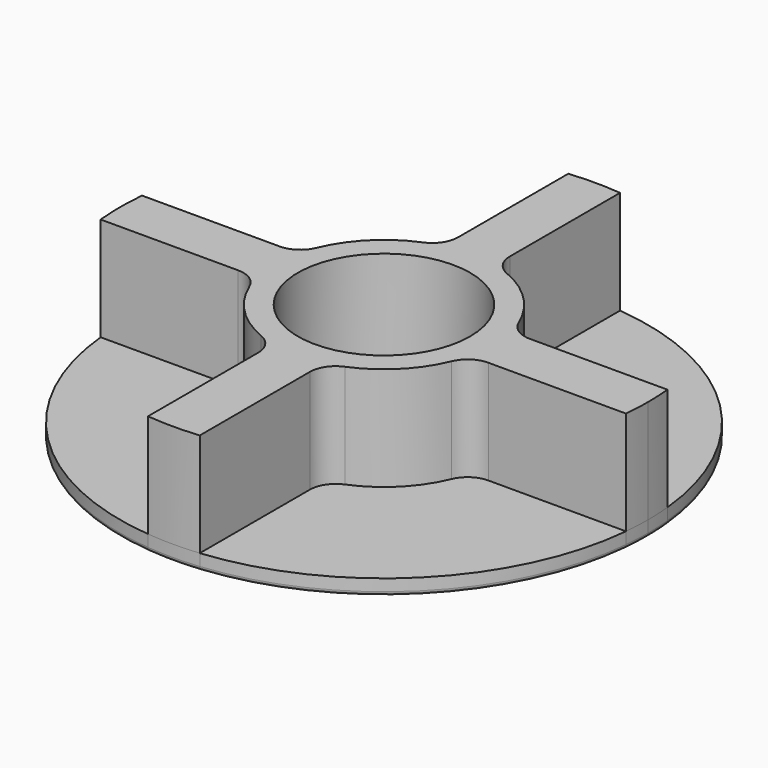
from build123d import *

# Parameters (mm, degrees)
F0_R     = 6.65
F0_R_2   = 1.8
F1_DEPTH = 1.2
F2_DEPTH = 8
F3_R     = 0.3


# Not quite as in the source:
# - a feature names something its author has since deleted; it is built from what else it names


with BuildPart() as f1:
    # F0 (on Top) → F1 (new body)
    with BuildSketch(Plane.XY):
        with BuildLine():
            Line((9.6529388756, 1.998378199), (20.2717385681, 1.998378199))
            ThreePointArc((20.2717385681, 1.998378199), (14.4037651328, 14.4037651328), (1.998378199, 20.2717385681))
            Line((1.998378199, 20.2717385681), (1.998378199, 9.6529388756))
            ThreePointArc((1.998378199, 9.6529388756), (2.3354389744, 8.5417984096), (3.2330113343, 7.8051798106))
            ThreePointArc((3.2330113343, 7.8051798106), (5.9738260003, 5.9738260003), (7.8051798106, 3.2330113343))
            ThreePointArc((7.8051798106, 3.2330113343), (8.5417984096, 2.3354389744), (9.6529388756, 1.998378199))
        make_face()
        with BuildLine():
            Line((-1.998378199, 9.6529388756), (-1.998378199, 20.2717385681))
            ThreePointArc((-1.998378199, 20.2717385681), (-14.4037651328, 14.4037651328), (-20.2717385681, 1.998378199))
            Line((-20.2717385681, 1.998378199), (-9.6529388756, 1.998378199))
            ThreePointArc((-9.6529388756, 1.998378199), (-8.5417984096, 2.3354389744), (-7.8051798106, 3.2330113343))
            ThreePointArc((-7.8051798106, 3.2330113343), (-5.9738260003, 5.9738260003), (-3.2330113343, 7.8051798106))
            ThreePointArc((-3.2330113343, 7.8051798106), (-2.3354389744, 8.5417984096), (-1.998378199, 9.6529388756))
        make_face()
        with BuildLine():
            ThreePointArc((-20.2717385681, -1.998378199), (-14.4037651328, -14.4037651328), (-1.998378199, -20.2717385681))
            Line((-1.998378199, -20.2717385681), (-1.998378199, -9.6529388756))
            ThreePointArc((-1.998378199, -9.6529388756), (-2.3354389744, -8.5417984096), (-3.2330113343, -7.8051798106))
            ThreePointArc((-3.2330113343, -7.8051798106), (-5.9738260003, -5.9738260003), (-7.8051798106, -3.2330113343))
            ThreePointArc((-7.8051798106, -3.2330113343), (-8.5417984096, -2.3354389744), (-9.6529388756, -1.998378199))
            Line((-9.6529388756, -1.998378199), (-20.2717385681, -1.998378199))
        make_face()
        with BuildLine():
            ThreePointArc((1.998378199, -20.2717385681), (14.4037651328, -14.4037651328), (20.2717385681, -1.998378199))
            Line((20.2717385681, -1.998378199), (9.6529388756, -1.998378199))
            ThreePointArc((9.6529388756, -1.998378199), (8.5417984096, -2.3354389744), (7.8051798106, -3.2330113343))
            ThreePointArc((7.8051798106, -3.2330113343), (5.9738260003, -5.9738260003), (3.2330113343, -7.8051798106))
            ThreePointArc((3.2330113343, -7.8051798106), (2.3354389744, -8.5417984096), (1.998378199, -9.6529388756))
            Line((1.998378199, -9.6529388756), (1.998378199, -20.2717385681))
        make_face()
        with BuildLine():
            ThreePointArc((20.2717385681, -1.998378199), (20.3454198117, -1.0003962634), (20.37, 0))
            ThreePointArc((20.37, 0), (20.3454198117, 1.0003962634), (20.2717385681, 1.998378199))
            Line((20.2717385681, 1.998378199), (9.6529388756, 1.998378199))
            ThreePointArc((9.6529388756, 1.998378199), (8.5417984096, 2.3354389744), (7.8051798106, 3.2330113343))
            ThreePointArc((7.8051798106, 3.2330113343), (5.9738260003, 5.9738260003), (3.2330113343, 7.8051798106))
            ThreePointArc((3.2330113343, 7.8051798106), (2.3354389744, 8.5417984096), (1.998378199, 9.6529388756))
            Line((1.998378199, 9.6529388756), (1.998378199, 20.2717385681))
            ThreePointArc((1.998378199, 20.2717385681), (0, 20.37), (-1.998378199, 20.2717385681))
            Line((-1.998378199, 20.2717385681), (-1.998378199, 9.6529388756))
            ThreePointArc((-1.998378199, 9.6529388756), (-2.3354389744, 8.5417984096), (-3.2330113343, 7.8051798106))
            ThreePointArc((-3.2330113343, 7.8051798106), (-5.9738260003, 5.9738260003), (-7.8051798106, 3.2330113343))
            ThreePointArc((-7.8051798106, 3.2330113343), (-8.5417984096, 2.3354389744), (-9.6529388756, 1.998378199))
            Line((-9.6529388756, 1.998378199), (-20.2717385681, 1.998378199))
            ThreePointArc((-20.2717385681, 1.998378199), (-20.37, 0), (-20.2717385681, -1.998378199))
            Line((-20.2717385681, -1.998378199), (-9.6529388756, -1.998378199))
            ThreePointArc((-9.6529388756, -1.998378199), (-8.5417984096, -2.3354389744), (-7.8051798106, -3.2330113343))
            ThreePointArc((-7.8051798106, -3.2330113343), (-5.9738260003, -5.9738260003), (-3.2330113343, -7.8051798106))
            ThreePointArc((-3.2330113343, -7.8051798106), (-2.3354389744, -8.5417984096), (-1.998378199, -9.6529388756))
            Line((-1.998378199, -9.6529388756), (-1.998378199, -20.2717385681))
            ThreePointArc((-1.998378199, -20.2717385681), (0, -20.37), (1.998378199, -20.2717385681))
            Line((1.998378199, -20.2717385681), (1.998378199, -9.6529388756))
            ThreePointArc((1.998378199, -9.6529388756), (2.3354389744, -8.5417984096), (3.2330113343, -7.8051798106))
            ThreePointArc((3.2330113343, -7.8051798106), (5.9738260003, -5.9738260003), (7.8051798106, -3.2330113343))
            ThreePointArc((7.8051798106, -3.2330113343), (8.5417984096, -2.3354389744), (9.6529388756, -1.998378199))
            Line((9.6529388756, -1.998378199), (20.2717385681, -1.998378199))
        make_face()
        Circle(F0_R, mode=Mode.SUBTRACT)
        Circle(F0_R)
        Circle(F0_R_2, mode=Mode.SUBTRACT)
    extrude(amount=-F1_DEPTH)

    # F0 (on Top) → F2 (join)
    with BuildSketch(Plane.XY):
        with BuildLine():
            ThreePointArc((20.2717385681, -1.998378199), (20.3454198117, -1.0003962634), (20.37, 0))
            ThreePointArc((20.37, 0), (20.3454198117, 1.0003962634), (20.2717385681, 1.998378199))
            Line((20.2717385681, 1.998378199), (9.6529388756, 1.998378199))
            ThreePointArc((9.6529388756, 1.998378199), (8.5417984096, 2.3354389744), (7.8051798106, 3.2330113343))
            ThreePointArc((7.8051798106, 3.2330113343), (5.9738260003, 5.9738260003), (3.2330113343, 7.8051798106))
            ThreePointArc((3.2330113343, 7.8051798106), (2.3354389744, 8.5417984096), (1.998378199, 9.6529388756))
            Line((1.998378199, 9.6529388756), (1.998378199, 20.2717385681))
            ThreePointArc((1.998378199, 20.2717385681), (0, 20.37), (-1.998378199, 20.2717385681))
            Line((-1.998378199, 20.2717385681), (-1.998378199, 9.6529388756))
            ThreePointArc((-1.998378199, 9.6529388756), (-2.3354389744, 8.5417984096), (-3.2330113343, 7.8051798106))
            ThreePointArc((-3.2330113343, 7.8051798106), (-5.9738260003, 5.9738260003), (-7.8051798106, 3.2330113343))
            ThreePointArc((-7.8051798106, 3.2330113343), (-8.5417984096, 2.3354389744), (-9.6529388756, 1.998378199))
            Line((-9.6529388756, 1.998378199), (-20.2717385681, 1.998378199))
            ThreePointArc((-20.2717385681, 1.998378199), (-20.37, 0), (-20.2717385681, -1.998378199))
            Line((-20.2717385681, -1.998378199), (-9.6529388756, -1.998378199))
            ThreePointArc((-9.6529388756, -1.998378199), (-8.5417984096, -2.3354389744), (-7.8051798106, -3.2330113343))
            ThreePointArc((-7.8051798106, -3.2330113343), (-5.9738260003, -5.9738260003), (-3.2330113343, -7.8051798106))
            ThreePointArc((-3.2330113343, -7.8051798106), (-2.3354389744, -8.5417984096), (-1.998378199, -9.6529388756))
            Line((-1.998378199, -9.6529388756), (-1.998378199, -20.2717385681))
            ThreePointArc((-1.998378199, -20.2717385681), (0, -20.37), (1.998378199, -20.2717385681))
            Line((1.998378199, -20.2717385681), (1.998378199, -9.6529388756))
            ThreePointArc((1.998378199, -9.6529388756), (2.3354389744, -8.5417984096), (3.2330113343, -7.8051798106))
            ThreePointArc((3.2330113343, -7.8051798106), (5.9738260003, -5.9738260003), (7.8051798106, -3.2330113343))
            ThreePointArc((7.8051798106, -3.2330113343), (8.5417984096, -2.3354389744), (9.6529388756, -1.998378199))
            Line((9.6529388756, -1.998378199), (20.2717385681, -1.998378199))
        make_face()
        Circle(F0_R, mode=Mode.SUBTRACT)
    extrude(amount=F2_DEPTH)

    # F3
    f3_edges = [f1.edges().sort_by_distance(p)[0] for p in [
        (-1.998378, -20.271739, -1.2),
    ]]
    fillet(f3_edges, radius=F3_R)


solid = f1.part
